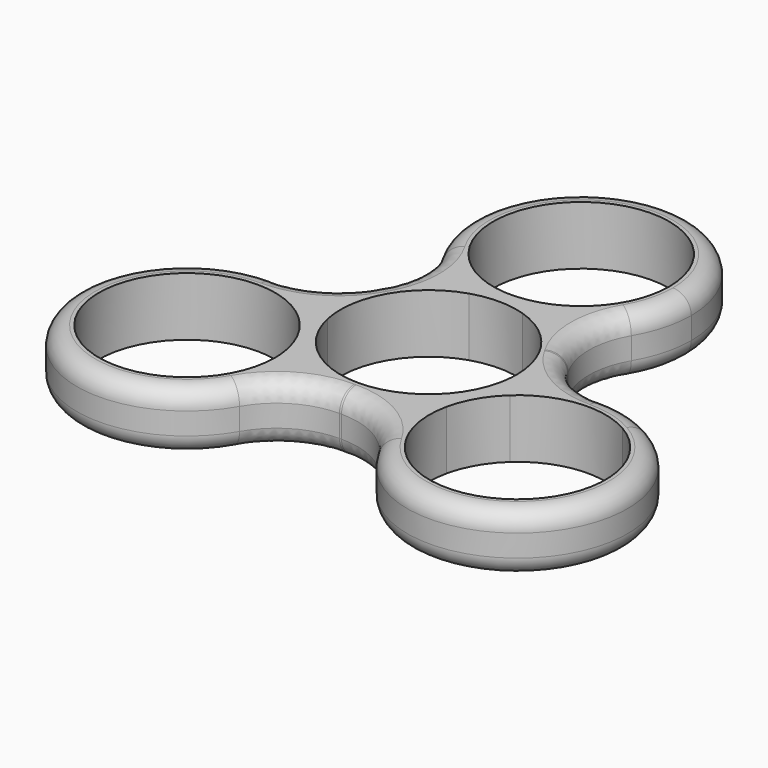
from build123d import *

# Parameters (mm, degrees)
F1_DEPTH = 8
F2_R     = 10.5869648701
F3_R     = 2.5


# Not quite as in the source:
# - a pattern or mirror of a feature is missing from the dataset's text; its kind, count and spacing are read off the source's solid


with BuildPart() as f1:
    # F0 (on Top) → F1 (new body)
    with BuildSketch(Plane.XY):
        with BuildLine():
            ThreePointArc((3.6157426173, 14.5576923077), (5.6039156019, 13.9138826331), (7.4833147735, 13))
            ThreePointArc((7.4833147735, 13), (12.9855635535, 18.4916620216), (15, 26))
            ThreePointArc((15, 26), (-7.5083379784, 38.9855635535), (-7.4833147735, 13))
            ThreePointArc((-7.4833147735, 13), (-5.6039156019, 13.9138826331), (-3.6157426173, 14.5576923077))
            ThreePointArc((-3.6157426173, 14.5576923077), (-7.0926401499, 35.6795896454), (12, 26))
            ThreePointArc((12, 26), (9.6795896454, 18.9073598501), (3.6157426173, 14.5576923077))
        make_face()
        with BuildLine():
            ThreePointArc((-11.7172004481, -2.589828886), (-10.3923048454, 6), (-3.6157426173, 11.4423076923))
            ThreePointArc((-3.6157426173, 11.4423076923), (-5.6039156019, 12.0861173669), (-7.4833147735, 13))
            ThreePointArc((-7.4833147735, 13), (-12.9903810568, 7.5), (-14.999987636, -0.0192593016))
            ThreePointArc((-14.999987636, -0.0192593016), (-13.2688424738, -1.1899254116), (-11.7172004481, -2.589828886))
        make_face()
        with BuildLine():
            ThreePointArc((-14.4152026676, -4.1475211937), (-14.8517336265, -2.1038080447), (-14.999987636, -0.0192593016))
            ThreePointArc((-14.999987636, -0.0192593016), (-35.5118537047, -20.4916589306), (-7.5166604984, -13))
            ThreePointArc((-7.5166604984, -13), (-7.5166635894, -12.9903703472), (-7.5166728624, -12.9807406984))
            ThreePointArc((-7.5166728624, -12.9807406984), (-9.2478180246, -11.8100745884), (-10.7994600503, -10.410171114))
            ThreePointArc((-10.7994600503, -10.410171114), (-10.5875698923, -11.697388273), (-10.5166604984, -13))
            ThreePointArc((-10.5166604984, -13), (-33.4988618708, -17.8364504562), (-14.4152026676, -4.1475211937))
        make_face()
        with BuildLine():
            ThreePointArc((-8.1014578308, -8.8524788063), (-10.3923048454, -6), (-11.7172004481, -2.589828886))
            ThreePointArc((-11.7172004481, -2.589828886), (-13.2688424738, -1.1899254116), (-14.999987636, -0.0192593016))
            ThreePointArc((-14.999987636, -0.0192593016), (-14.8517336265, -2.1038080447), (-14.4152026676, -4.1475211937))
            ThreePointArc((-14.4152026676, -4.1475211937), (-12.124355653, -7), (-10.7994600503, -10.410171114))
            ThreePointArc((-10.7994600503, -10.410171114), (-9.2478180246, -11.8100745884), (-7.5166728624, -12.9807406984))
            ThreePointArc((-7.5166728624, -12.9807406984), (-7.6649268719, -10.8961919553), (-8.1014578308, -8.8524788063))
        make_face()
        with BuildLine():
            ThreePointArc((14.999987636, -0.0192593016), (13.2688424738, -1.1899254116), (11.7172004481, -2.589828886))
            ThreePointArc((11.7172004481, -2.589828886), (10.3923048454, -6), (8.1014578308, -8.8524788063))
            ThreePointArc((8.1014578308, -8.8524788063), (7.6649268719, -10.8961919553), (7.5166728624, -12.9807406984))
            ThreePointArc((7.5166728624, -12.9807406984), (9.2478180246, -11.8100745884), (10.7994600503, -10.410171114))
            ThreePointArc((10.7994600503, -10.410171114), (12.124355653, -7), (14.4152026676, -4.1475211937))
            ThreePointArc((14.4152026676, -4.1475211937), (14.8517336265, -2.1038080447), (14.999987636, -0.0192593016))
        make_face()
        with BuildLine():
            ThreePointArc((7.5166728624, -12.9807406984), (7.6649268719, -10.8961919553), (8.1014578308, -8.8524788063))
            ThreePointArc((8.1014578308, -8.8524788063), (0, -12), (-8.1014578308, -8.8524788063))
            ThreePointArc((-8.1014578308, -8.8524788063), (-7.6649268719, -10.8961919553), (-7.5166728624, -12.9807406984))
            ThreePointArc((-7.5166728624, -12.9807406984), (0, -15), (7.5166728624, -12.9807406984))
        make_face()
        with BuildLine():
            ThreePointArc((3.6157426173, 11.4423076923), (9.6795896454, 7.0926401499), (12, 0))
            ThreePointArc((12, 0), (11.9290906061, -1.302611727), (11.7172004481, -2.589828886))
            ThreePointArc((11.7172004481, -2.589828886), (13.2688424738, -1.1899254116), (14.999987636, -0.0192593016))
            ThreePointArc((14.999987636, -0.0192593016), (14.999996909, -0.0096296528), (15, 0))
            ThreePointArc((15, 0), (12.9855635535, 7.5083379784), (7.4833147735, 13))
            ThreePointArc((7.4833147735, 13), (5.6039156019, 12.0861173669), (3.6157426173, 11.4423076923))
        make_face()
        with BuildLine():
            ThreePointArc((-3.6157426173, 11.4423076923), (0, 12), (3.6157426173, 11.4423076923))
            ThreePointArc((3.6157426173, 11.4423076923), (5.6039156019, 12.0861173669), (7.4833147735, 13))
            ThreePointArc((7.4833147735, 13), (5.6039156019, 13.9138826331), (3.6157426173, 14.5576923077))
            ThreePointArc((3.6157426173, 14.5576923077), (0, 14), (-3.6157426173, 14.5576923077))
            ThreePointArc((-3.6157426173, 14.5576923077), (-5.6039156019, 13.9138826331), (-7.4833147735, 13))
            ThreePointArc((-7.4833147735, 13), (-5.6039156019, 12.0861173669), (-3.6157426173, 11.4423076923))
        make_face()
    extrude(amount=F1_DEPTH)

    # F1_copies: F1 across plane


with BuildPart() as f1_1:
    add(f1.part)
    add(f1.part.mirror(Plane(origin=(0, 0, 0), x_dir=(-0.8660254038, -0.5, 0), z_dir=(0.5, -0.8660254038, 0))))

    # F2
    f2_edges = [f1_1.edges().sort_by_distance(p)[0] for p in [
        (7.483315, 13, 4),
        (14.999988, -0.019259, 4),
        (-7.516673, -12.980741, 4),
        (-7.483315, 13, 4),
        (-14.999988, -0.019259, 4),
        (7.516673, -12.980741, 4),
    ]]
    fillet(f2_edges, radius=F2_R)

    # F3
    f3_edges = [f1_1.edges().sort_by_distance(p)[0] for p in [
        (-35.507042, -20.5, 8),
        (35.507042, -20.5, 8),
        (0, 41, 8),
        (0, 41, 0),
        (-11.451474, 13, 0),
        (-35.507042, -20.5, 0),
        (35.507042, -20.5, 0),
        (11.451474, 13, 0),
        (12.990381, 7.5, 0),
        (-12.990381, 7.5, 0),
        (16.984067, 3.417267, 0),
        (-16.984067, 3.417267, 0),
        (5.532593, -16.417267, 0),
        (-5.532593, -16.417267, 0),
        (0, -15, 0),
        (11.451474, 13, 8),
        (-11.451474, 13, 8),
        (12.990381, 7.5, 8),
        (-12.990381, 7.5, 8),
        (16.984067, 3.417267, 8),
        (-16.984067, 3.417267, 8),
        (5.532593, -16.417267, 8),
        (-5.532593, -16.417267, 8),
        (0, -15, 8),
    ]]
    fillet(f3_edges, radius=F3_R)


solid = f1_1.part
